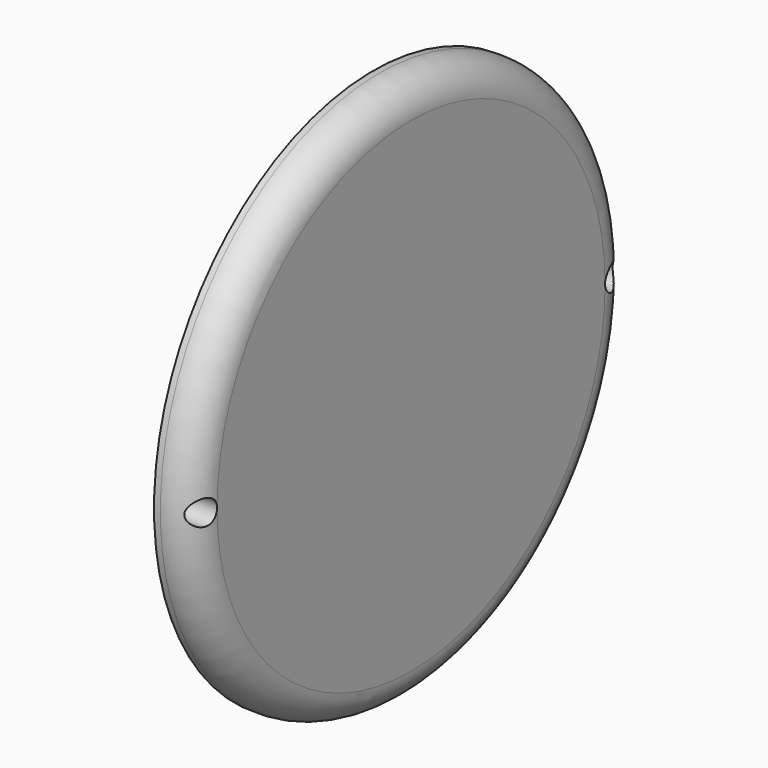
from build123d import *

# Parameters (mm, degrees)
F0_R     = 43.5
F0_R_2   = 2
F1_DEPTH = 6


# Not quite as in the source:
# - a fillet or chamfer that OpenCascade refuses, or shapes differently, is made with other operations: its cross-section is extruded or revolved along the edge and cut away or added


with BuildPart() as f1:
    # F0 (on Right) → F1 (new body)
    with BuildSketch(Plane.YZ):
        Circle(F0_R)
        with Locations((-40.5, 0)):
            Circle(F0_R_2, mode=Mode.SUBTRACT)
        with Locations((40.5, 0)):
            Circle(F0_R_2, mode=Mode.SUBTRACT)
    extrude(amount=-F1_DEPTH)

    # F2: fillet of radius 5 on 1 edges, made by hand

    # F2_s1 → F2_t2 (revolve, cut)
    with BuildSketch(Plane.XY):
        with BuildLine():
            ThreePointArc((-5, 43.5), (-1.4644660941, 42.0355339059), (0, 38.5))
            Line((0, 38.5), (0, 43.5))
            Line((0, 43.5), (-5, 43.5))
        make_face()
    revolve(axis=Axis((0, 0, 0), (1, 0, 0)), mode=Mode.SUBTRACT)


solid = f1.part
